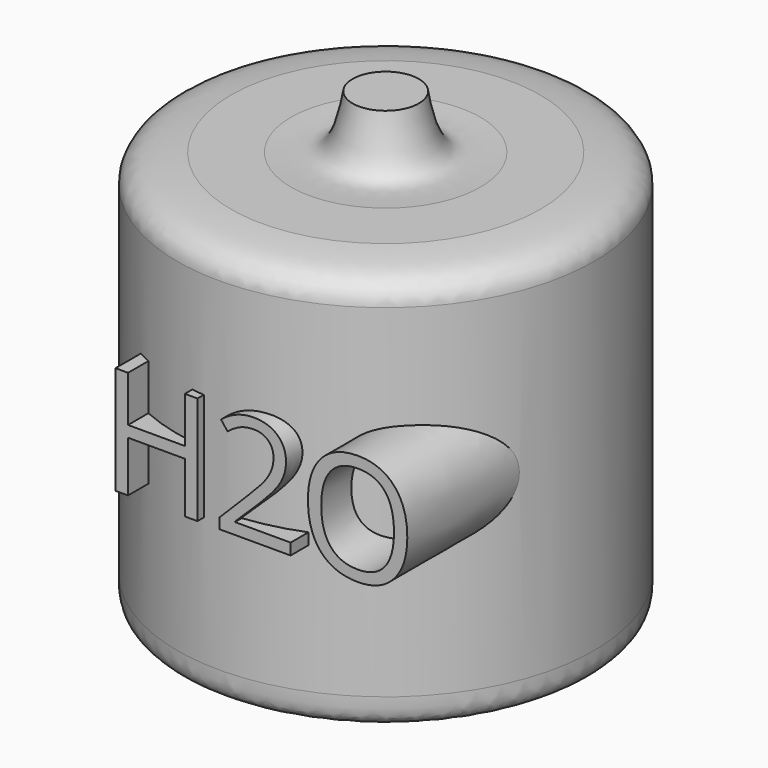
from build123d import *

# Parameters (mm, degrees)
F3_TEXT_SIZE = 18.1628856808


# Not quite as in the source:
# - Text() gives the source's letters only with a copy of the font that has no kerning and outlines rounded to 1/6400 em; it was checked with that copy


with BuildPart() as f1:
    # F0 (on Front) → F1 (revolve)
    with BuildSketch(Plane.XZ):
        with BuildLine():
            Line((-22.3724655807, 0), (0, 0))
            Line((0, 0), (0, 54.9831725657))
            Line((0, 54.9831725657), (-3.9815395139, 54.9831725657))
            add(Edge.make_bspline(
                [(-11.3758295774, 48.5368743539), (-9.6510130221, 48.5368743539), (-6.5634997353, 47.7033232285), (-4.6861645794, 51.0633189838), (-4.2277063321, 53.6076772881), (-3.9815395139, 54.9831725657)],
                knots=[0, 0, 0, 0, 0.360351496, 0.6582432995, 1, 1, 1, 1], degree=3))
            Line((-11.3758295774, 48.5368743539), (-18.5805223882, 48.5368743539))
            add(Edge.make_bspline(
                [(-25.026826188, 45.1241247356), (-25.026826188, 46.0295345731), (-23.8604496207, 48.0252682466), (-20.6035543011, 48.3598452602), (-18.5805223882, 48.5368743539)],
                knots=[0, 0, 0, 0, 0.414766212, 1, 1, 1, 1], degree=3))
            Line((-25.026826188, 45.1241247356), (-25.026826188, 3.9815404452))
            add(Edge.make_bspline(
                [(-22.3724655807, 0), (-23.2909657363, 0.414869438), (-25.0968918164, 1.2260436907), (-25.026826188, 3.0770011316), (-25.026826188, 3.9815404452)],
                knots=[0, 0, 0, 0, 0.5115133318, 1, 1, 1, 1], degree=3))
        make_face()
    revolve(axis=Axis((0, 0, 27.4915862828), (0, 0, -1)))

    # F3 (on offset) → F4 (join, up to the next surface of F1)
    with BuildSketch(Plane.XZ.offset(25.908)):
        with Locations((-13.5041810572, 19.4587856531)):
            Text('H2O', F3_TEXT_SIZE, font='Open Sans', text_align=(TextAlign.LEFT, TextAlign.BOTTOM))
    extrude(until=Until.NEXT, dir=(0, 1, 0))


solid = f1.part
